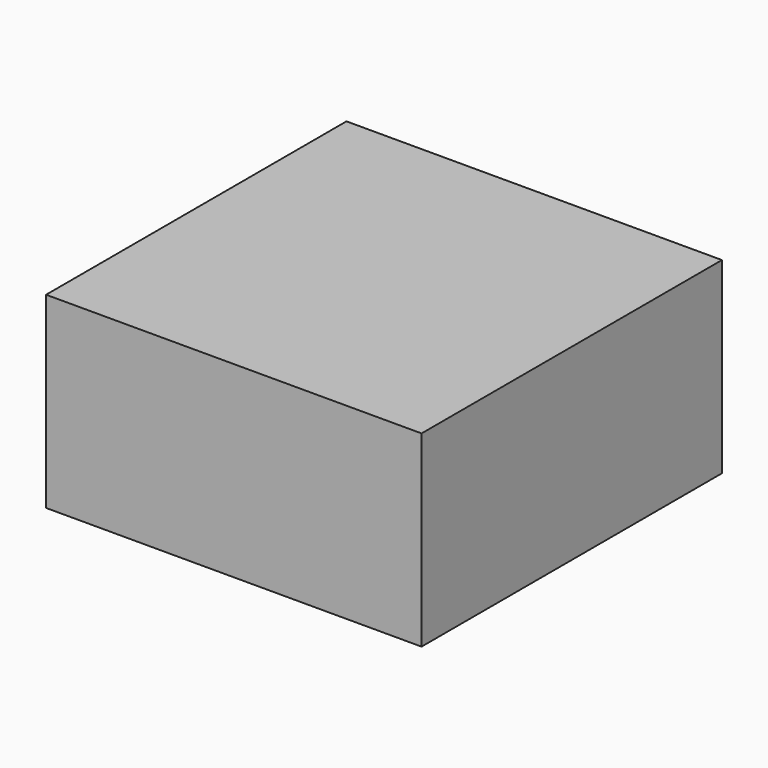
from build123d import *

# Parameters (mm, degrees)
F1_W     = 100
F1_H     = 50
F2_DEPTH = 100


# Not quite as in the source:
# - the program builds the solid bodies; features that only make, move or delete a surface that nothing else refers to are left out


with BuildPart() as f2:
    # F1 (on Right) → F2 (new body)
    with BuildSketch(Plane.YZ):
        with Locations((-2.6405041123, -12.6058591495)):
            Rectangle(F1_W, F1_H)
    extrude(amount=F2_DEPTH)


solid = f2.part
